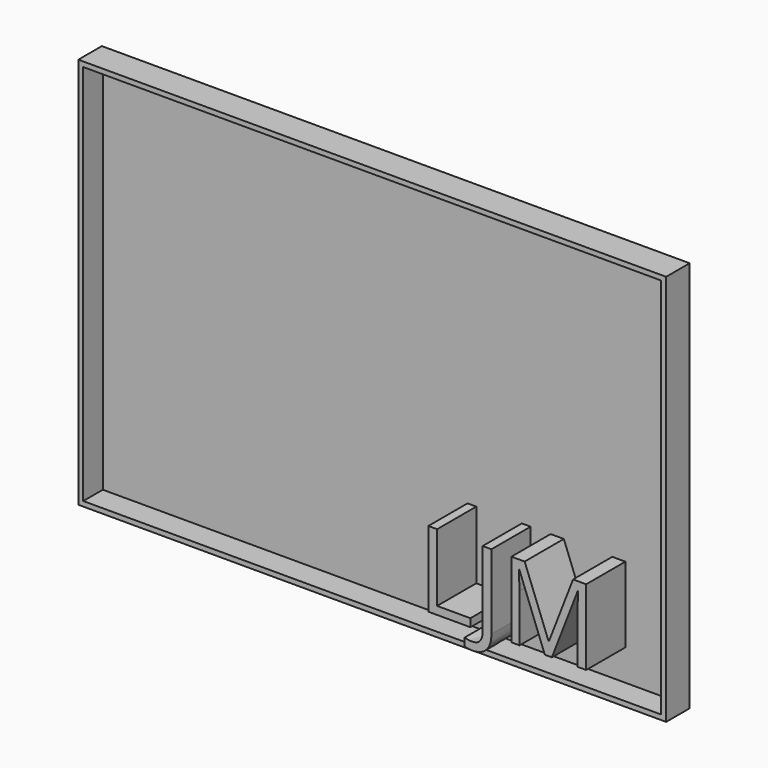
from build123d import *

# Parameters (mm, degrees)
F1_DEPTH     = 15
F2_T         = -2.5
F3_TEXT_SIZE = 53.9535604831
F4_DEPTH     = 25
F5_R         = 20
F6_DEPTH     = 70


# Not quite as in the source:
# - Text() gives the source's letters only with a copy of the font that has no kerning and outlines rounded to 1/6400 em; it was checked with that copy


with BuildPart() as f1:
    # F0 (on Front) → F1 (new body)
    with BuildSketch(Plane.XZ):
        Polygon((0, 100), (-150, 100), (-150, -100), (150, -100), (150, 100), align=None)
    extrude(amount=F1_DEPTH)

    # F2
    f2_openings = [f1.faces().sort_by_distance(p)[0] for p in [
        (0, -15, 0),
    ]]
    offset(amount=F2_T, openings=f2_openings)

    # F3 (on face) → F4 (join)
    with BuildSketch(Plane.XZ.offset(2.5)):
        with Locations((33.329628408, -81.6136077046)):
            Text('LJM', F3_TEXT_SIZE, font='Open Sans', text_align=(TextAlign.LEFT, TextAlign.BOTTOM))
    extrude(amount=F4_DEPTH)

    # F5 (on face) → F6 (join)
    with BuildSketch(Plane(origin=(0, 0, 0), x_dir=(-1, 0, 0), z_dir=(0, 1, 0))):
        Circle(F5_R)
    extrude(amount=F6_DEPTH)


solid = f1.part
